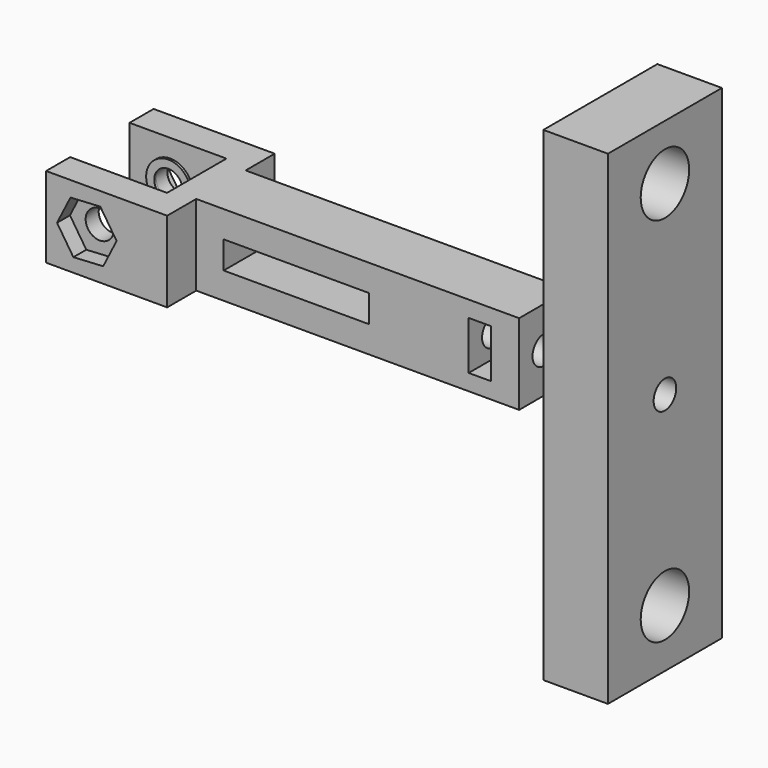
from build123d import *

# Parameters (mm, degrees)
F0_W      = 40
F0_H      = 3.825
F1_DEPTH  = 10
F2_R      = 1.75
F3_DEPTH  = 16.651
F4_W      = 18
F4_H      = 3.4
F4_W_2    = 2.75
F4_H_2    = 6
F5_DEPTH  = 12.151
F6_R      = 1.75
F7_DEPTH  = 15
F10_DEPTH = 2
F11_W     = 17.65
F11_H     = 60
F12_DEPTH = 8
F13_R     = 1.75
F14_DEPTH = 70.001
F15_R     = 2.75
F15_R_2   = 1.75
F16_DEPTH = 0.3
F17_R     = 1.75
F18_DEPTH = 2
F19_R     = 3.75
F20_DEPTH = 15


# Not quite as in the source:
# - a pattern or mirror of a feature is missing from the dataset's text; its kind, count and spacing are read off the source's solid


with BuildPart() as f1:
    # F0 (on Top) → F1 (new body)
    with BuildSketch(Plane.XY):
        Polygon((0, -3.825), (0, 0), (-3, 0), (-3, -4.6), (-15, -4.6), (-15, -8.325), (0, -8.325), align=None)
        Polygon((-3, 0), (0, 0), (0, 3.825), (0, 8.325), (-15, 8.325), (-15, 4.6), (-3, 4.6), align=None)
        with Locations((20, 1.9125)):
            Rectangle(F0_W, F0_H)
        with Locations((20, -1.9125)):
            Rectangle(F0_W, F0_H)
    extrude(amount=F1_DEPTH)

    # F2 (on face) → F3 (cut, through all)
    with BuildSketch(Plane.XZ.offset(8.325)):
        with Locations((-9.9527407438, 5)):
            Circle(F2_R)
    extrude(amount=-F3_DEPTH, mode=Mode.SUBTRACT)

    # F4 (on face) → F5 (cut, through all)
    with BuildSketch(Plane.XZ.offset(3.825)):
        with Locations((12.4002694301, 5)):
            Rectangle(F4_W, F4_H)
        with Locations((35.125, 5)):
            Rectangle(F4_W_2, F4_H_2)
    extrude(amount=-F5_DEPTH, mode=Mode.SUBTRACT)

    # F6 (on face) → F7 (cut)
    with BuildSketch(Plane.YZ.offset(40)):
        with Locations((0, 5)):
            Circle(F6_R)
    extrude(amount=-F7_DEPTH, mode=Mode.SUBTRACT)

    # F15 (on face) → F16 (join)
    with BuildSketch(Plane.XZ.offset(-4.6)):
        with Locations((-9.9527407438, 5)):
            Circle(F15_R)
        with Locations((-9.9527407438, 5)):
            Circle(F15_R_2, mode=Mode.SUBTRACT)
    f16 = extrude(amount=F16_DEPTH)

    # F16_copies: F16 across plane
    add(f16.mirror(Plane(origin=(0, 0, 0), x_dir=(0, 0, -1), z_dir=(0, -1, 0))))

    # F17 (on face) → F18 (cut)
    with BuildSketch(Plane.XZ.offset(8.325)):
        Polygon((-7.9284293953, 1.9088033227), (-6.2635302189, 5.2075067143), (-8.2878415673, 8.2987033916), (-11.9770520922, 8.0911966773), (-13.6419512686, 4.7924932857), (-11.6176399202, 1.7012966084), align=None)
        with Locations((-9.9527407438, 5)):
            Circle(F17_R, mode=Mode.SUBTRACT)
    f18 = extrude(amount=-F18_DEPTH, mode=Mode.SUBTRACT)

    # F18_copies: F18 across plane
    add(f18.mirror(Plane.ZX), mode=Mode.SUBTRACT)


with BuildPart() as f10:
    # F9 (on offset) → F10 (new body)
    with BuildSketch(Plane.YZ.offset(45)):
        Polygon((3.825, 0), (3.825, 10), (3.825, 19.8484882712), (-3.825, 19.8484882712), (-3.825, 10), (-3.825, 0), (-3.825, -10.1515117288), (3.825, -10.1515117288), align=None)
    extrude(amount=F10_DEPTH)

    # F11 (on face) → F12 (join)
    with BuildSketch(Plane.YZ.offset(47)):
        with Locations((0, 4.8484882712)):
            Rectangle(F11_W, F11_H)
    extrude(amount=F12_DEPTH)

    # F13 (on face) → F14 (cut, through all)
    with BuildSketch(Plane.YZ.offset(55)):
        with Locations((0, 5)):
            Circle(F13_R)
    extrude(amount=-F14_DEPTH, mode=Mode.SUBTRACT)

    # F19 (on face) → F20 (cut)
    with BuildSketch(Plane(origin=(47, 0, 0), x_dir=(0, -1, 0), z_dir=(-1, 0, 0))):
        with Locations((0, 28)):
            Circle(F19_R)
        with Locations((0, -18)):
            Circle(F19_R)
    extrude(amount=-F20_DEPTH, mode=Mode.SUBTRACT)


solid = Compound([f1.part, f10.part])
